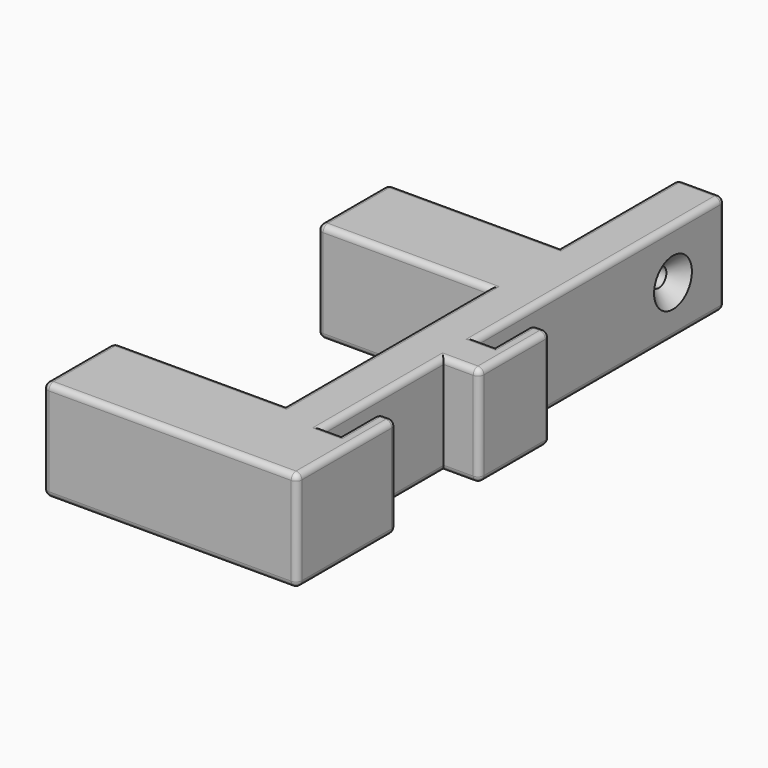
from build123d import *

# Parameters (mm, degrees)
F1_DEPTH       = 17
F3_D           = 3.2
F3_CSINK_D     = 8
F3_CSINK_ANGLE = 90
F4_R           = 1
F5_T1_DEPTH    = 15
F5_S5_W        = 1
F5_S5_H        = 1
F5_T6_DEPTH    = 1
F5_S11_W       = 1
F5_S11_H       = 1
F5_T12_DEPTH   = 1
F5_S17_W       = 1
F5_S17_H       = 1
F5_T18_DEPTH   = 1
F5_S23_W       = 1
F5_S23_H       = 1
F5_T24_DEPTH   = 1
F5_S29_W       = 1
F5_S29_H       = 1
F5_T30_DEPTH   = 1
F5_S35_W       = 1
F5_S35_H       = 1
F5_T36_DEPTH   = 1
F5_S41_W       = 1
F5_S41_H       = 1
F5_T42_DEPTH   = 1
F5_S47_W       = 1
F5_S47_H       = 1
F5_T48_DEPTH   = 1
F5_S53_W       = 1
F5_S53_H       = 1
F5_T54_DEPTH   = 1
F5_S59_W       = 1
F5_S59_H       = 1
F5_T60_DEPTH   = 1
F6_T1_DEPTH    = 15
F6_S5_W        = 1
F6_S5_H        = 1
F6_T6_DEPTH    = 1
F6_S11_W       = 1
F6_S11_H       = 1
F6_T12_DEPTH   = 1
F6_S17_W       = 1
F6_S17_H       = 1
F6_T18_DEPTH   = 1
F6_S23_W       = 1
F6_S23_H       = 1
F6_T24_DEPTH   = 1
F6_S29_W       = 1
F6_S29_H       = 1
F6_T30_DEPTH   = 1
F6_S35_W       = 1
F6_S35_H       = 1
F6_T36_DEPTH   = 1
F6_S41_W       = 1
F6_S41_H       = 1
F6_T42_DEPTH   = 1
F6_S47_W       = 1
F6_S47_H       = 1
F6_T48_DEPTH   = 1
F6_S53_W       = 1
F6_S53_H       = 1
F6_T54_DEPTH   = 1
F6_S59_W       = 1
F6_S59_H       = 1
F6_T60_DEPTH   = 1
F6_S65_W       = 1
F6_S65_H       = 1
F6_T66_DEPTH   = 1
F6_S71_W       = 1
F6_S71_H       = 1
F6_T72_DEPTH   = 1
F6_S77_W       = 1
F6_S77_H       = 1
F6_T78_DEPTH   = 1
F6_S83_W       = 1
F6_S83_H       = 1
F6_T84_DEPTH   = 1


# Not quite as in the source:
# - a fillet or chamfer that OpenCascade refuses, or shapes differently, is made with other operations: its cross-section is extruded or revolved along the edge and cut away or added


with BuildPart() as f1:
    # F0 (on Top) → F1 (new body)
    with BuildSketch(Plane.XY):
        Polygon((-29, 21.5), (0, 21.5), (0, -21.5), (-29, -21.5), (-29, -36.5), (14, -36.5), (14, -15.5), (11, -15.5), (11, -23.5), (8, -23.5), (8, 2), (14, 2), (14, 17), (11, 17), (11, 9), (8, 9), (8, 61.5), (0, 61.5), (0, 36.5), (-29, 36.5), align=None)
    extrude(amount=F1_DEPTH)

    # F3 (through all)
    with Locations(Plane.YZ.offset(8)):
        with Locations((50.5, 8.5)):
            CounterSinkHole(F3_D / 2, F3_CSINK_D / 2, counter_sink_angle=F3_CSINK_ANGLE)

    # F4
    f4_edges = [f1.edges().sort_by_distance(p)[0] for p in [
        (-14.5, 21.5, 17),
        (0, 0, 17),
        (-14.5, -21.5, 17),
        (-29, -29, 17),
        (-7.5, -36.5, 17),
        (14, -26, 17),
        (12.5, -15.5, 17),
        (11, -19.5, 17),
        (9.5, -23.5, 17),
        (8, -10.75, 17),
        (11, 2, 17),
        (14, 9.5, 17),
        (12.5, 17, 17),
        (11, 13, 17),
        (9.5, 9, 17),
        (8, 35.25, 17),
        (4, 61.5, 17),
        (0, 49, 17),
        (-14.5, 36.5, 17),
        (-29, 29, 17),
        (-14.5, 21.5, 0),
        (0, 0, 0),
        (-14.5, -21.5, 0),
        (-29, -29, 0),
        (-7.5, -36.5, 0),
        (14, -26, 0),
        (12.5, -15.5, 0),
        (11, -19.5, 0),
        (9.5, -23.5, 0),
        (8, -10.75, 0),
        (11, 2, 0),
        (14, 9.5, 0),
        (12.5, 17, 0),
        (11, 13, 0),
        (9.5, 9, 0),
        (8, 35.25, 0),
        (4, 61.5, 0),
        (0, 49, 0),
        (-14.5, 36.5, 0),
        (-29, 29, 0),
    ]]
    fillet(f4_edges, radius=F4_R)

    # F5: fillet of radius 1 on 5 edges, made by hand

    # F5_s2 → F5_t1 (cut)
    with BuildSketch(Plane.XY.offset(1)):
        with BuildLine():
            ThreePointArc((0, 60.5), (0.2928932188, 61.2071067812), (1, 61.5))
            Line((1, 61.5), (0, 61.5))
            Line((0, 61.5), (0, 60.5))
        make_face()
        with BuildLine():
            ThreePointArc((-29, 35.5), (-28.7071067812, 36.2071067812), (-28, 36.5))
            Line((-28, 36.5), (-29, 36.5))
            Line((-29, 36.5), (-29, 35.5))
        make_face()
        with BuildLine():
            ThreePointArc((-28, 21.5), (-28.7071067812, 21.7928932188), (-29, 22.5))
            Line((-29, 22.5), (-29, 21.5))
            Line((-29, 21.5), (-28, 21.5))
        make_face()
        with BuildLine():
            ThreePointArc((-28, -21.5), (-28.7071067812, -21.7928932188), (-29, -22.5))
            Line((-29, -22.5), (-29, -21.5))
            Line((-29, -21.5), (-28, -21.5))
        make_face()
        with BuildLine():
            ThreePointArc((-29, -35.5), (-28.7071067812, -36.2071067812), (-28, -36.5))
            Line((-28, -36.5), (-29, -36.5))
            Line((-29, -36.5), (-29, -35.5))
        make_face()
    extrude(amount=F5_T1_DEPTH, mode=Mode.SUBTRACT)


with BuildPart() as f5_tool4:
    # F5_s5 → F5_t6 (new body)
    with BuildSketch(Plane.YZ.offset(-28)):
        with Locations((-36, 0.5)):
            Rectangle(F5_S5_W, F5_S5_H)
    extrude(amount=-F5_T6_DEPTH)

    # F5_s7 → F5_t8 (revolve, cut)
    with BuildSketch(Plane(origin=(-28, -35.5, 1), x_dir=(0, 0.7071067812, 0.7071067812), z_dir=(0, -0.7071067812, 0.7071067812))):
        with BuildLine():
            ThreePointArc((0, -1), (1, 0), (0, 1))
            Line((0, 1), (0, -1))
        make_face()
    revolve(axis=Axis((-28, -35.5, 1), (-1, 0, 0)), mode=Mode.SUBTRACT)


with BuildPart() as f1_1:
    add(f1.part)

    # F5_t3: cut F5_tool4
    add(f5_tool4.part, mode=Mode.SUBTRACT)


with BuildPart() as f5_tool10:
    # F5_s11 → F5_t12 (new body)
    with BuildSketch(Plane.YZ.offset(-28)):
        with Locations((-36, 16.5)):
            Rectangle(F5_S11_W, F5_S11_H)
    extrude(amount=-F5_T12_DEPTH)

    # F5_s13 → F5_t14 (revolve, cut)
    with BuildSketch(Plane(origin=(-28, -35.5, 16), x_dir=(0, 0.7071067812, -0.7071067812), z_dir=(0, 0.7071067812, 0.7071067812))):
        with BuildLine():
            ThreePointArc((0, -1), (1, 0), (0, 1))
            Line((0, 1), (0, -1))
        make_face()
    revolve(axis=Axis((-28, -35.5, 16), (-1, 0, 0)), mode=Mode.SUBTRACT)


with BuildPart() as f1_2:
    add(f1_1.part)

    # F5_t9: cut F5_tool10
    add(f5_tool10.part, mode=Mode.SUBTRACT)


with BuildPart() as f5_tool16:
    # F5_s17 → F5_t18 (new body)
    with BuildSketch(Plane.XZ.offset(22.5)):
        with Locations((-28.5, 0.5)):
            Rectangle(F5_S17_W, F5_S17_H)
    extrude(amount=-F5_T18_DEPTH)

    # F5_s19 → F5_t20 (revolve, cut)
    with BuildSketch(Plane(origin=(-28, -22.5, 1), x_dir=(0.7071067812, 0, 0.7071067812), z_dir=(-0.7071067812, 0, 0.7071067812))):
        with BuildLine():
            ThreePointArc((0, -1), (1, 0), (0, 1))
            Line((0, 1), (0, -1))
        make_face()
    revolve(axis=Axis((-28, -22.5, 1), (0, 1, 0)), mode=Mode.SUBTRACT)


with BuildPart() as f1_3:
    add(f1_2.part)

    # F5_t15: cut F5_tool16
    add(f5_tool16.part, mode=Mode.SUBTRACT)


with BuildPart() as f5_tool22:
    # F5_s23 → F5_t24 (new body)
    with BuildSketch(Plane.XZ.offset(22.5)):
        with Locations((-28.5, 16.5)):
            Rectangle(F5_S23_W, F5_S23_H)
    extrude(amount=-F5_T24_DEPTH)

    # F5_s25 → F5_t26 (revolve, cut)
    with BuildSketch(Plane(origin=(-28, -22.5, 16), x_dir=(0.7071067812, 0, -0.7071067812), z_dir=(0.7071067812, 0, 0.7071067812))):
        with BuildLine():
            ThreePointArc((0, -1), (1, 0), (0, 1))
            Line((0, 1), (0, -1))
        make_face()
    revolve(axis=Axis((-28, -22.5, 16), (0, 1, 0)), mode=Mode.SUBTRACT)


with BuildPart() as f1_4:
    add(f1_3.part)

    # F5_t21: cut F5_tool22
    add(f5_tool22.part, mode=Mode.SUBTRACT)


with BuildPart() as f5_tool28:
    # F5_s29 → F5_t30 (new body)
    with BuildSketch(Plane.XZ.offset(-22.5)):
        with Locations((-28.5, 0.5)):
            Rectangle(F5_S29_W, F5_S29_H)
    extrude(amount=F5_T30_DEPTH)

    # F5_s31 → F5_t32 (revolve, cut)
    with BuildSketch(Plane(origin=(-28, 22.5, 1), x_dir=(0.7071067812, 0, 0.7071067812), z_dir=(0.7071067812, 0, -0.7071067812))):
        with BuildLine():
            ThreePointArc((0, -1), (1, 0), (0, 1))
            Line((0, 1), (0, -1))
        make_face()
    revolve(axis=Axis((-28, 22.5, 1), (0, -1, 0)), mode=Mode.SUBTRACT)


with BuildPart() as f1_5:
    add(f1_4.part)

    # F5_t27: cut F5_tool28
    add(f5_tool28.part, mode=Mode.SUBTRACT)


with BuildPart() as f5_tool34:
    # F5_s35 → F5_t36 (new body)
    with BuildSketch(Plane.XZ.offset(-22.5)):
        with Locations((-28.5, 16.5)):
            Rectangle(F5_S35_W, F5_S35_H)
    extrude(amount=F5_T36_DEPTH)

    # F5_s37 → F5_t38 (revolve, cut)
    with BuildSketch(Plane(origin=(-28, 22.5, 16), x_dir=(0.7071067812, 0, -0.7071067812), z_dir=(-0.7071067812, 0, -0.7071067812))):
        with BuildLine():
            ThreePointArc((0, -1), (1, 0), (0, 1))
            Line((0, 1), (0, -1))
        make_face()
    revolve(axis=Axis((-28, 22.5, 16), (0, -1, 0)), mode=Mode.SUBTRACT)


with BuildPart() as f1_6:
    add(f1_5.part)

    # F5_t33: cut F5_tool34
    add(f5_tool34.part, mode=Mode.SUBTRACT)


with BuildPart() as f5_tool40:
    # F5_s41 → F5_t42 (new body)
    with BuildSketch(Plane.YZ.offset(-28)):
        with Locations((36, 0.5)):
            Rectangle(F5_S41_W, F5_S41_H)
    extrude(amount=-F5_T42_DEPTH)

    # F5_s43 → F5_t44 (revolve, cut)
    with BuildSketch(Plane(origin=(-28, 35.5, 1), x_dir=(0, -0.7071067812, 0.7071067812), z_dir=(0, -0.7071067812, -0.7071067812))):
        with BuildLine():
            ThreePointArc((0, -1), (1, 0), (0, 1))
            Line((0, 1), (0, -1))
        make_face()
    revolve(axis=Axis((-28, 35.5, 1), (-1, 0, 0)), mode=Mode.SUBTRACT)


with BuildPart() as f1_7:
    add(f1_6.part)

    # F5_t39: cut F5_tool40
    add(f5_tool40.part, mode=Mode.SUBTRACT)


with BuildPart() as f5_tool46:
    # F5_s47 → F5_t48 (new body)
    with BuildSketch(Plane.YZ.offset(-28)):
        with Locations((36, 16.5)):
            Rectangle(F5_S47_W, F5_S47_H)
    extrude(amount=-F5_T48_DEPTH)

    # F5_s49 → F5_t50 (revolve, cut)
    with BuildSketch(Plane(origin=(-28, 35.5, 16), x_dir=(0, -0.7071067812, -0.7071067812), z_dir=(0, 0.7071067812, -0.7071067812))):
        with BuildLine():
            ThreePointArc((0, -1), (1, 0), (0, 1))
            Line((0, 1), (0, -1))
        make_face()
    revolve(axis=Axis((-28, 35.5, 16), (-1, 0, 0)), mode=Mode.SUBTRACT)


with BuildPart() as f1_8:
    add(f1_7.part)

    # F5_t45: cut F5_tool46
    add(f5_tool46.part, mode=Mode.SUBTRACT)


with BuildPart() as f5_tool52:
    # F5_s53 → F5_t54 (new body)
    with BuildSketch(Plane.YZ.offset(1)):
        with Locations((61, 0.5)):
            Rectangle(F5_S53_W, F5_S53_H)
    extrude(amount=-F5_T54_DEPTH)

    # F5_s55 → F5_t56 (revolve, cut)
    with BuildSketch(Plane(origin=(1, 60.5, 1), x_dir=(0, -0.7071067812, 0.7071067812), z_dir=(0, -0.7071067812, -0.7071067812))):
        with BuildLine():
            ThreePointArc((0, -1), (1, 0), (0, 1))
            Line((0, 1), (0, -1))
        make_face()
    revolve(axis=Axis((1, 60.5, 1), (-1, 0, 0)), mode=Mode.SUBTRACT)


with BuildPart() as f1_9:
    add(f1_8.part)

    # F5_t51: cut F5_tool52
    add(f5_tool52.part, mode=Mode.SUBTRACT)


with BuildPart() as f5_tool58:
    # F5_s59 → F5_t60 (new body)
    with BuildSketch(Plane.YZ.offset(1)):
        with Locations((61, 16.5)):
            Rectangle(F5_S59_W, F5_S59_H)
    extrude(amount=-F5_T60_DEPTH)

    # F5_s61 → F5_t62 (revolve, cut)
    with BuildSketch(Plane(origin=(1, 60.5, 16), x_dir=(0, -0.7071067812, -0.7071067812), z_dir=(0, 0.7071067812, -0.7071067812))):
        with BuildLine():
            ThreePointArc((0, -1), (1, 0), (0, 1))
            Line((0, 1), (0, -1))
        make_face()
    revolve(axis=Axis((1, 60.5, 16), (-1, 0, 0)), mode=Mode.SUBTRACT)


with BuildPart() as f1_10:
    add(f1_9.part)

    # F5_t57: cut F5_tool58
    add(f5_tool58.part, mode=Mode.SUBTRACT)

    # F6: fillet of radius 1 on 7 edges, made by hand

    # F6_s2 → F6_t1 (cut)
    with BuildSketch(Plane.XY.offset(1)):
        with BuildLine():
            ThreePointArc((11, 16), (11.2928932188, 16.7071067812), (12, 17))
            Line((12, 17), (11, 17))
            Line((11, 17), (11, 16))
        make_face()
        with BuildLine():
            ThreePointArc((13, 17), (13.7071067812, 16.7071067812), (14, 16))
            Line((14, 16), (14, 17))
            Line((14, 17), (13, 17))
        make_face()
        with BuildLine():
            ThreePointArc((12, -15.5), (11.2928932188, -15.7928932188), (11, -16.5))
            Line((11, -16.5), (11, -15.5))
            Line((11, -15.5), (12, -15.5))
        make_face()
        with BuildLine():
            ThreePointArc((14, -16.5), (13.7071067812, -15.7928932188), (13, -15.5))
            Line((13, -15.5), (14, -15.5))
            Line((14, -15.5), (14, -16.5))
        make_face()
        with BuildLine():
            ThreePointArc((14, 3), (13.7071067812, 2.2928932188), (13, 2))
            Line((13, 2), (14, 2))
            Line((14, 2), (14, 3))
        make_face()
        with BuildLine():
            ThreePointArc((13, -36.5), (13.7071067812, -36.2071067812), (14, -35.5))
            Line((14, -35.5), (14, -36.5))
            Line((14, -36.5), (13, -36.5))
        make_face()
        with BuildLine():
            ThreePointArc((7, 61.5), (7.7071067812, 61.2071067812), (8, 60.5))
            Line((8, 60.5), (8, 61.5))
            Line((8, 61.5), (7, 61.5))
        make_face()
    extrude(amount=F6_T1_DEPTH, mode=Mode.SUBTRACT)


with BuildPart() as f6_tool4:
    # F6_s5 → F6_t6 (new body)
    with BuildSketch(Plane.XZ.offset(-60.5)):
        with Locations((7.5, 0.5)):
            Rectangle(F6_S5_W, F6_S5_H)
    extrude(amount=-F6_T6_DEPTH)

    # F6_s7 → F6_t8 (revolve, cut)
    with BuildSketch(Plane(origin=(7, 60.5, 1), x_dir=(-0.7071067812, 0, 0.7071067812), z_dir=(-0.7071067812, 0, -0.7071067812))):
        with BuildLine():
            ThreePointArc((0, -1), (1, 0), (0, 1))
            Line((0, 1), (0, -1))
        make_face()
    revolve(axis=Axis((7, 60.5, 1), (0, 1, 0)), mode=Mode.SUBTRACT)


with BuildPart() as f1_11:
    add(f1_10.part)

    # F6_t3: cut F6_tool4
    add(f6_tool4.part, mode=Mode.SUBTRACT)


with BuildPart() as f6_tool10:
    # F6_s11 → F6_t12 (new body)
    with BuildSketch(Plane.XZ.offset(-60.5)):
        with Locations((7.5, 16.5)):
            Rectangle(F6_S11_W, F6_S11_H)
    extrude(amount=-F6_T12_DEPTH)

    # F6_s13 → F6_t14 (revolve, cut)
    with BuildSketch(Plane(origin=(7, 60.5, 16), x_dir=(-0.7071067812, 0, -0.7071067812), z_dir=(0.7071067812, 0, -0.7071067812))):
        with BuildLine():
            ThreePointArc((0, -1), (1, 0), (0, 1))
            Line((0, 1), (0, -1))
        make_face()
    revolve(axis=Axis((7, 60.5, 16), (0, 1, 0)), mode=Mode.SUBTRACT)


with BuildPart() as f1_12:
    add(f1_11.part)

    # F6_t9: cut F6_tool10
    add(f6_tool10.part, mode=Mode.SUBTRACT)


with BuildPart() as f6_tool16:
    # F6_s17 → F6_t18 (new body)
    with BuildSketch(Plane.XZ.offset(35.5)):
        with Locations((13.5, 0.5)):
            Rectangle(F6_S17_W, F6_S17_H)
    extrude(amount=F6_T18_DEPTH)

    # F6_s19 → F6_t20 (revolve, cut)
    with BuildSketch(Plane(origin=(13, -35.5, 1), x_dir=(-0.7071067812, 0, 0.7071067812), z_dir=(0.7071067812, 0, 0.7071067812))):
        with BuildLine():
            ThreePointArc((0, -1), (1, 0), (0, 1))
            Line((0, 1), (0, -1))
        make_face()
    revolve(axis=Axis((13, -35.5, 1), (0, -1, 0)), mode=Mode.SUBTRACT)


with BuildPart() as f1_13:
    add(f1_12.part)

    # F6_t15: cut F6_tool16
    add(f6_tool16.part, mode=Mode.SUBTRACT)


with BuildPart() as f6_tool22:
    # F6_s23 → F6_t24 (new body)
    with BuildSketch(Plane.XZ.offset(35.5)):
        with Locations((13.5, 16.5)):
            Rectangle(F6_S23_W, F6_S23_H)
    extrude(amount=F6_T24_DEPTH)

    # F6_s25 → F6_t26 (revolve, cut)
    with BuildSketch(Plane(origin=(13, -35.5, 16), x_dir=(-0.7071067812, 0, -0.7071067812), z_dir=(-0.7071067812, 0, 0.7071067812))):
        with BuildLine():
            ThreePointArc((0, -1), (1, 0), (0, 1))
            Line((0, 1), (0, -1))
        make_face()
    revolve(axis=Axis((13, -35.5, 16), (0, -1, 0)), mode=Mode.SUBTRACT)


with BuildPart() as f1_14:
    add(f1_13.part)

    # F6_t21: cut F6_tool22
    add(f6_tool22.part, mode=Mode.SUBTRACT)


with BuildPart() as f6_tool28:
    # F6_s29 → F6_t30 (new body)
    with BuildSketch(Plane.YZ.offset(13)):
        with Locations((2.5, 0.5)):
            Rectangle(F6_S29_W, F6_S29_H)
    extrude(amount=F6_T30_DEPTH)

    # F6_s31 → F6_t32 (revolve, cut)
    with BuildSketch(Plane(origin=(13, 3, 1), x_dir=(0, 0.7071067812, 0.7071067812), z_dir=(0, 0.7071067812, -0.7071067812))):
        with BuildLine():
            ThreePointArc((0, -1), (1, 0), (0, 1))
            Line((0, 1), (0, -1))
        make_face()
    revolve(axis=Axis((13, 3, 1), (1, 0, 0)), mode=Mode.SUBTRACT)


with BuildPart() as f1_15:
    add(f1_14.part)

    # F6_t27: cut F6_tool28
    add(f6_tool28.part, mode=Mode.SUBTRACT)


with BuildPart() as f6_tool34:
    # F6_s35 → F6_t36 (new body)
    with BuildSketch(Plane.YZ.offset(13)):
        with Locations((2.5, 16.5)):
            Rectangle(F6_S35_W, F6_S35_H)
    extrude(amount=F6_T36_DEPTH)

    # F6_s37 → F6_t38 (revolve, cut)
    with BuildSketch(Plane(origin=(13, 3, 16), x_dir=(0, 0.7071067812, -0.7071067812), z_dir=(0, -0.7071067812, -0.7071067812))):
        with BuildLine():
            ThreePointArc((0, -1), (1, 0), (0, 1))
            Line((0, 1), (0, -1))
        make_face()
    revolve(axis=Axis((13, 3, 16), (1, 0, 0)), mode=Mode.SUBTRACT)


with BuildPart() as f1_16:
    add(f1_15.part)

    # F6_t33: cut F6_tool34
    add(f6_tool34.part, mode=Mode.SUBTRACT)


with BuildPart() as f6_tool40:
    # F6_s41 → F6_t42 (new body)
    with BuildSketch(Plane.YZ.offset(13)):
        with Locations((-16, 0.5)):
            Rectangle(F6_S41_W, F6_S41_H)
    extrude(amount=F6_T42_DEPTH)

    # F6_s43 → F6_t44 (revolve, cut)
    with BuildSketch(Plane(origin=(13, -16.5, 1), x_dir=(0, -0.7071067812, 0.7071067812), z_dir=(0, 0.7071067812, 0.7071067812))):
        with BuildLine():
            ThreePointArc((0, -1), (1, 0), (0, 1))
            Line((0, 1), (0, -1))
        make_face()
    revolve(axis=Axis((13, -16.5, 1), (1, 0, 0)), mode=Mode.SUBTRACT)


with BuildPart() as f1_17:
    add(f1_16.part)

    # F6_t39: cut F6_tool40
    add(f6_tool40.part, mode=Mode.SUBTRACT)


with BuildPart() as f6_tool46:
    # F6_s47 → F6_t48 (new body)
    with BuildSketch(Plane.YZ.offset(13)):
        with Locations((-16, 16.5)):
            Rectangle(F6_S47_W, F6_S47_H)
    extrude(amount=F6_T48_DEPTH)

    # F6_s49 → F6_t50 (revolve, cut)
    with BuildSketch(Plane(origin=(13, -16.5, 16), x_dir=(0, -0.7071067812, -0.7071067812), z_dir=(0, -0.7071067812, 0.7071067812))):
        with BuildLine():
            ThreePointArc((0, -1), (1, 0), (0, 1))
            Line((0, 1), (0, -1))
        make_face()
    revolve(axis=Axis((13, -16.5, 16), (1, 0, 0)), mode=Mode.SUBTRACT)


with BuildPart() as f1_18:
    add(f1_17.part)

    # F6_t45: cut F6_tool46
    add(f6_tool46.part, mode=Mode.SUBTRACT)


with BuildPart() as f6_tool52:
    # F6_s53 → F6_t54 (new body)
    with BuildSketch(Plane.XZ.offset(16.5)):
        with Locations((11.5, 0.5)):
            Rectangle(F6_S53_W, F6_S53_H)
    extrude(amount=-F6_T54_DEPTH)

    # F6_s55 → F6_t56 (revolve, cut)
    with BuildSketch(Plane(origin=(12, -16.5, 1), x_dir=(0.7071067812, 0, 0.7071067812), z_dir=(-0.7071067812, 0, 0.7071067812))):
        with BuildLine():
            ThreePointArc((0, -1), (1, 0), (0, 1))
            Line((0, 1), (0, -1))
        make_face()
    revolve(axis=Axis((12, -16.5, 1), (0, 1, 0)), mode=Mode.SUBTRACT)


with BuildPart() as f1_19:
    add(f1_18.part)

    # F6_t51: cut F6_tool52
    add(f6_tool52.part, mode=Mode.SUBTRACT)


with BuildPart() as f6_tool58:
    # F6_s59 → F6_t60 (new body)
    with BuildSketch(Plane.XZ.offset(16.5)):
        with Locations((11.5, 16.5)):
            Rectangle(F6_S59_W, F6_S59_H)
    extrude(amount=-F6_T60_DEPTH)

    # F6_s61 → F6_t62 (revolve, cut)
    with BuildSketch(Plane(origin=(12, -16.5, 16), x_dir=(0.7071067812, 0, -0.7071067812), z_dir=(0.7071067812, 0, 0.7071067812))):
        with BuildLine():
            ThreePointArc((0, -1), (1, 0), (0, 1))
            Line((0, 1), (0, -1))
        make_face()
    revolve(axis=Axis((12, -16.5, 16), (0, 1, 0)), mode=Mode.SUBTRACT)


with BuildPart() as f1_20:
    add(f1_19.part)

    # F6_t57: cut F6_tool58
    add(f6_tool58.part, mode=Mode.SUBTRACT)


with BuildPart() as f6_tool64:
    # F6_s65 → F6_t66 (new body)
    with BuildSketch(Plane.XZ.offset(-16)):
        with Locations((13.5, 0.5)):
            Rectangle(F6_S65_W, F6_S65_H)
    extrude(amount=-F6_T66_DEPTH)

    # F6_s67 → F6_t68 (revolve, cut)
    with BuildSketch(Plane(origin=(13, 16, 1), x_dir=(-0.7071067812, 0, 0.7071067812), z_dir=(-0.7071067812, 0, -0.7071067812))):
        with BuildLine():
            ThreePointArc((0, -1), (1, 0), (0, 1))
            Line((0, 1), (0, -1))
        make_face()
    revolve(axis=Axis((13, 16, 1), (0, 1, 0)), mode=Mode.SUBTRACT)


with BuildPart() as f1_21:
    add(f1_20.part)

    # F6_t63: cut F6_tool64
    add(f6_tool64.part, mode=Mode.SUBTRACT)


with BuildPart() as f6_tool70:
    # F6_s71 → F6_t72 (new body)
    with BuildSketch(Plane.XZ.offset(-16)):
        with Locations((13.5, 16.5)):
            Rectangle(F6_S71_W, F6_S71_H)
    extrude(amount=-F6_T72_DEPTH)

    # F6_s73 → F6_t74 (revolve, cut)
    with BuildSketch(Plane(origin=(13, 16, 16), x_dir=(-0.7071067812, 0, -0.7071067812), z_dir=(0.7071067812, 0, -0.7071067812))):
        with BuildLine():
            ThreePointArc((0, -1), (1, 0), (0, 1))
            Line((0, 1), (0, -1))
        make_face()
    revolve(axis=Axis((13, 16, 16), (0, 1, 0)), mode=Mode.SUBTRACT)


with BuildPart() as f1_22:
    add(f1_21.part)

    # F6_t69: cut F6_tool70
    add(f6_tool70.part, mode=Mode.SUBTRACT)


with BuildPart() as f6_tool76:
    # F6_s77 → F6_t78 (new body)
    with BuildSketch(Plane.YZ.offset(12)):
        with Locations((16.5, 0.5)):
            Rectangle(F6_S77_W, F6_S77_H)
    extrude(amount=-F6_T78_DEPTH)

    # F6_s79 → F6_t80 (revolve, cut)
    with BuildSketch(Plane(origin=(12, 16, 1), x_dir=(0, -0.7071067812, 0.7071067812), z_dir=(0, -0.7071067812, -0.7071067812))):
        with BuildLine():
            ThreePointArc((0, -1), (1, 0), (0, 1))
            Line((0, 1), (0, -1))
        make_face()
    revolve(axis=Axis((12, 16, 1), (-1, 0, 0)), mode=Mode.SUBTRACT)


with BuildPart() as f1_23:
    add(f1_22.part)

    # F6_t75: cut F6_tool76
    add(f6_tool76.part, mode=Mode.SUBTRACT)


with BuildPart() as f6_tool82:
    # F6_s83 → F6_t84 (new body)
    with BuildSketch(Plane.YZ.offset(12)):
        with Locations((16.5, 16.5)):
            Rectangle(F6_S83_W, F6_S83_H)
    extrude(amount=-F6_T84_DEPTH)

    # F6_s85 → F6_t86 (revolve, cut)
    with BuildSketch(Plane(origin=(12, 16, 16), x_dir=(0, -0.7071067812, -0.7071067812), z_dir=(0, 0.7071067812, -0.7071067812))):
        with BuildLine():
            ThreePointArc((0, -1), (1, 0), (0, 1))
            Line((0, 1), (0, -1))
        make_face()
    revolve(axis=Axis((12, 16, 16), (-1, 0, 0)), mode=Mode.SUBTRACT)


with BuildPart() as f1_24:
    add(f1_23.part)

    # F6_t81: cut F6_tool82
    add(f6_tool82.part, mode=Mode.SUBTRACT)


solid = f1_24.part
